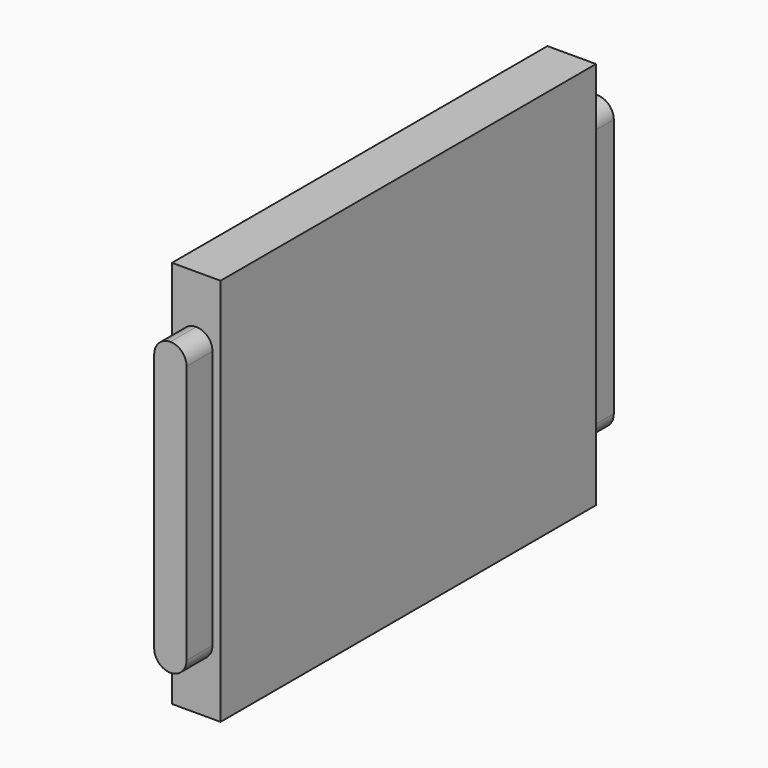
from build123d import *

# Parameters (mm, degrees)
F0_W     = 19.05
F0_H     = 184.15
F1_DEPTH = 152.4
F2_W     = 12.7
F2_H     = 114.3
F3_DEPTH = 12.7
F4_W     = 12.7
F4_H     = 114.3
F5_DEPTH = 12.7
F6_R     = 6.34999


# Not quite as in the source:
# - a fillet or chamfer is up to 0.001 mm smaller than in the source, because OpenCascade refuses the exact size


with BuildPart() as f1:
    # F0 (on Top) → F1 (new body)
    with BuildSketch(Plane.XY):
        Rectangle(F0_W, F0_H)
    extrude(amount=-F1_DEPTH)

    # F2 (on face) → F3 (join)
    with BuildSketch(Plane.XZ.offset(92.075)):
        with Locations((0, -76.2)):
            Rectangle(F2_W, F2_H)
    extrude(amount=F3_DEPTH)

    # F4 (on face) → F5 (join)
    with BuildSketch(Plane(origin=(0, 92.075, 0), x_dir=(-1, 0, 0), z_dir=(0, 1, 0))):
        with Locations((0, -76.2)):
            Rectangle(F4_W, F4_H)
    extrude(amount=F5_DEPTH)

    # F6 (radius 6.35 in the source; OpenCascade refuses exactly that, so slightly less here)
    f6_edges = [f1.edges().sort_by_distance(p)[0] for p in [
        (6.35, 98.425, -19.05),
        (-6.35, 98.425, -19.05),
        (-6.35, 98.425, -133.35),
        (6.35, 98.425, -133.35),
        (-6.35, -98.425, -19.05),
        (6.35, -98.425, -19.05),
        (-6.35, -98.425, -133.35),
        (6.35, -98.425, -133.35),
    ]]
    fillet(f6_edges, radius=F6_R)


solid = f1.part
